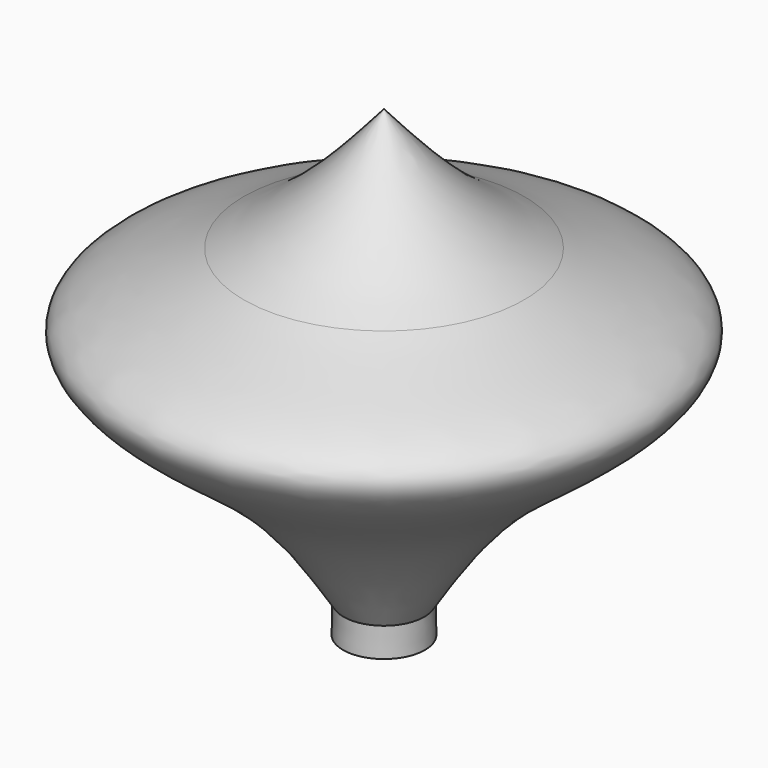
from build123d import *

# Parameters (mm, degrees)
F2_DEPTH = 18.796
F3_DEPTH = 25.4


with BuildPart() as f1:
    # F0 (on Front) → F1 (revolve)
    with BuildSketch(Plane.XZ):
        Polygon((-3.1376469415, 26.0953336054), (0, 26.0995179415), (0, 36.9026255262), (-3.1376469415, 36.9026255262), align=None)
    revolve(axis=Axis((0, 0, 11.1243847059), (0, 0, -1)))

    # F2 (cut): a face of the model
    f2_faces = [f1.faces().sort_by_distance(p)[0] for p in [
        (0, 0, 36.9026255262),
    ]]
    extrude(f2_faces, amount=-F2_DEPTH, mode=Mode.SUBTRACT)


with BuildPart() as f1b:
    # F0 (on Front) → F1, piece 2 (revolve)
    with BuildSketch(Plane.XZ):
        with BuildLine():
            Line((0, 0), (0, 16.8363694102))
            add(Edge.make_bspline(
                [(0, 16.8363694102), (-3.474241628, 12.8596777576), (-6.9484832559, 8.882986105), (-12.1888345, 6.1778346719)],
                knots=[0, 0, 0, 0, 0.2663691303, 0.2663691303, 0.2663691303, 0.2663691303], degree=3))
            add(Edge.make_bspline(
                [(-12.1888345, 6.1778346719), (-16.7755084747, 3.810121689), (-29.2204528037, 0.8901901789), (-10.2664559429, -10.2391590135), (-5.7337599776, -17.3964564632), (-3.5136023088, -20.9021689447)],
                knots=[0.2663691303, 0.2663691303, 0.2663691303, 0.2663691303, 0.4995115859, 0.7548560064, 1, 1, 1, 1], degree=3))
            Line((-3.5136023088, -20.9021689447), (-3.5625977907, -23.424660787))
            Line((-3.5625977907, -23.424660787), (-1.886081649, -23.4572245063))
            Line((-1.886081649, -23.4572245063), (0, -23.4938587097))
            Line((0, -23.4938587097), (0, -20.6523918138))
            Line((0, -20.6523918138), (0, -15.5456149951))
            Line((0, -15.5456149951), (0, -3.8507485297))
            Line((0, -3.8507485297), (0, 0))
        make_face()
        Polygon((0, -23.4938587097), (-1.886081649, -23.4572245063), (-1.886081649, -25.1011773944), (0, -25.1011773944), align=None)
    revolve(axis=Axis((0, 0, 11.1243847059), (0, 0, -1)))

    # F3 (cut): a face of the model
    f3_faces = [f1b.faces().sort_by_distance(p)[0] for p in [
        (0, 0, -25.1011773944),
    ]]
    extrude(f3_faces, amount=-F3_DEPTH, mode=Mode.SUBTRACT)


solid = f1b.part
